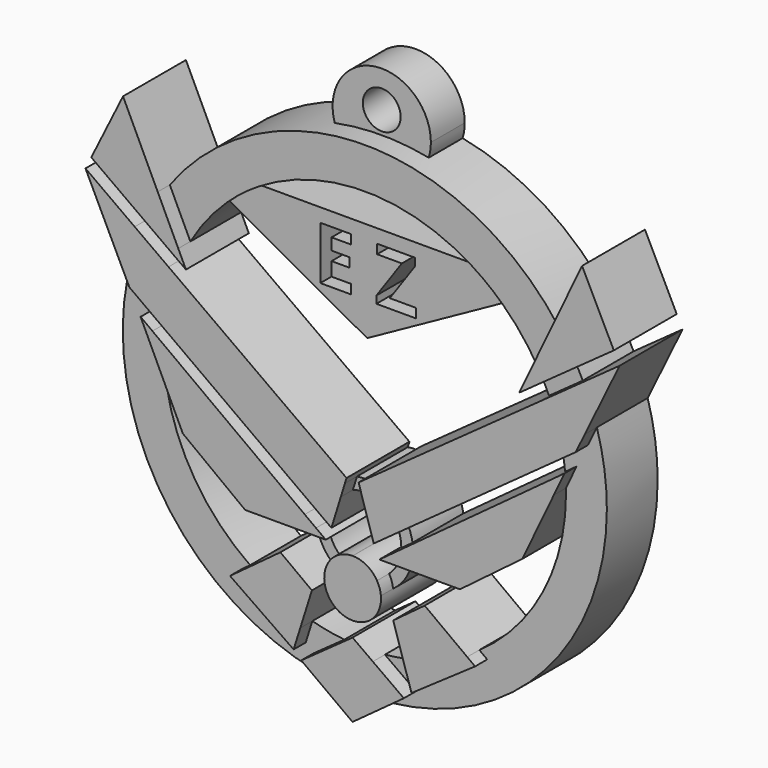
from build123d import *

# Parameters (mm, degrees)
F1_DEPTH = 1.524
F2_DEPTH = 0.254
F3_DEPTH = 5.08
F4_DEPTH = 5.08
F0_R     = 1.5875
F5_DEPTH = 5.08
F6_DEPTH = 1.524


# Not quite as in the source:
# - after a boolean that leaves OpenCascade's solid faulty, fix() repairs it
# - ends of sketch curves that miss each other by under 0.0002 mm in the source are joined
# - a feature names something its author has since deleted; it is built from what else it names


with BuildPart() as f1:
    # F0 (on Front) → F1 (new body)
    with BuildSketch(Plane.XZ):
        with BuildLine():
            Line((-29.3892786764, 17.9176513211), (-25.2442078939, 14.9377645788))
            ThreePointArc((-25.2442078939, 14.9377645788), (-24.5641804468, 16.083185728), (-23.8106040275, 17.1816162074))
            Line((-23.8106040275, 17.1816162074), (-26.7234016986, 23.3000394668))
            Line((-26.7234016986, 23.3000394668), (-29.3892786764, 17.9176513211))
        make_face()
        with BuildLine():
            ThreePointArc((-23.8106040275, 17.1816162074), (-24.5641804468, 16.083185728), (-25.2442078939, 14.9377645788))
            Line((-25.2442078939, 14.9377645788), (-22.4329405216, 12.9167476141))
            ThreePointArc((-22.4329405216, 12.9167476141), (-22.2620008814, 13.2378637775), (-22.084188419, 13.5552258408))
            Line((-22.084188419, 13.5552258408), (-23.8106040275, 17.1816162074))
        make_face()
        with BuildLine():
            ThreePointArc((-22.084188419, 13.5552258408), (-22.2620008814, 13.2378637775), (-22.4329405216, 12.9167476141))
            Line((-22.4329405216, 12.9167476141), (-21.4406050886, 12.2033587829))
            Line((-21.4406050886, 12.2033587829), (-22.084188419, 13.5552258408))
        make_face()
        with BuildLine():
            ThreePointArc((-25.7430354928, 13.9707437059), (-26.401196412, 12.4512059686), (-26.9335086266, 10.8831452437))
            Line((-26.9335086266, 10.8831452437), (-26.1902267417, 9.3535226814))
            Line((-26.1902267417, 9.3535226814), (-24.1110498022, 7.849707391))
            ThreePointArc((-24.1110498022, 7.849707391), (-23.6368154324, 9.9281026338), (-22.9046772821, 11.9302511677))
            Line((-22.9046772821, 11.9302511677), (-25.7430354928, 13.9707437059))
        make_face()
        with BuildLine():
            Line((-29.8784934974, 16.9437198329), (-26.9335086266, 10.8831452437))
            ThreePointArc((-26.9335086266, 10.8831452437), (-26.401196412, 12.4512059686), (-25.7430354928, 13.9707437059))
            Line((-25.7430354928, 13.9707437059), (-29.8784934974, 16.9437198329))
        make_face()
        with BuildLine():
            ThreePointArc((-22.9046772821, 11.9302511677), (-23.6368154324, 9.9281026338), (-24.1110498022, 7.849707391))
            Line((-24.1110498022, 7.849707391), (-11.1208236013, -1.5457896518))
            ThreePointArc((-11.1208236013, -1.5457896518), (-9.886951438, -0.0314606923), (-8.0895618793, 0.7334075888))
            Line((-8.0895618793, 0.7334075888), (-7.9511925062, 1.180207713))
            Line((-7.9511925062, 1.180207713), (-22.9046772821, 11.9302511677))
        make_face()
        with BuildLine():
            ThreePointArc((-8.0895618793, 0.7334075888), (-9.886951438, -0.0314606923), (-11.1208236013, -1.5457896518))
            Line((-11.1208236013, -1.5457896518), (-10.2965646805, -2.1419549635))
            ThreePointArc((-10.2965646805, -2.1419549635), (-9.5580579554, -1.0532702062), (-8.4321576163, -0.3728474624))
            Line((-8.4321576163, -0.3728474624), (-8.0895618793, 0.7334075888))
        make_face()
        with BuildLine():
            ThreePointArc((-8.4321576163, -0.3728474624), (-9.5580579554, -1.0532702062), (-10.2965646805, -2.1419549635))
            Line((-10.2965646805, -2.1419549635), (-9.2209577128, -2.9199138634))
            Line((-9.2209577128, -2.9199138634), (-8.4321576163, -0.3728474624))
        make_face()
        with BuildLine():
            ThreePointArc((-24.2536135862, 6.7439211254), (-24.3005868215, 6.1366695), (-24.3256460235, 5.5281195367))
            Line((-24.3256460235, 5.5281195367), (-21.7045924914, 0))
            Line((-21.7045924914, 0), (-16.4677212918, -3.9508687748))
            Line((-16.4677212918, -3.9508687748), (-11.4556599361, -3.9508687748))
            ThreePointArc((-11.4556599361, -3.9508687748), (-11.5106514951, -3.3027910164), (-11.4616861743, -2.6542301095))
            Line((-11.4616861743, -2.6542301095), (-24.2536135862, 6.7439211254))
        make_face()
        with BuildLine():
            ThreePointArc((-17.0661091722, -8.7456602207), (-14.5563398729, -10.1858082926), (-11.8376665018, -11.1766581835))
            Line((-11.8376665018, -11.1766581835), (-10.8605655167, -8.0768892639))
            Line((-10.8605655167, -8.0768892639), (-13.5054501714, -6.1196745536))
            Line((-13.5054501714, -6.1196745536), (-17.0661091722, -8.7456602207))
        make_face()
        with BuildLine():
            Line((-7.4453192851, -10.4538336357), (-9.147168429, -11.6738428354))
            ThreePointArc((-9.147168429, -11.6738428354), (-7.4437042085, -11.7611295901), (-5.7401185733, -11.676245483))
            Line((-5.7401185733, -11.676245483), (-7.4453192851, -10.4538336357))
        make_face()
        with BuildLine():
            Line((-9.147168429, -11.6738428354), (-11.7522682075, -13.541367761))
            Line((-11.7522682075, -13.541367761), (-9.6607773298, -15.0707744806))
            ThreePointArc((-9.6607773298, -15.0707744806), (-7.4477977116, -15.1933278019), (-5.2346278181, -15.0742600496))
            Line((-5.2346278181, -15.0742600496), (-3.1383703627, -13.541367761))
            Line((-3.1383703627, -13.541367761), (-5.7401185733, -11.676245483))
            ThreePointArc((-5.7401185733, -11.676245483), (-7.4437042085, -11.7611295901), (-9.147168429, -11.6738428354))
        make_face()
        with BuildLine():
            Line((-12.3945986384, -12.9434775331), (-11.8376665018, -11.1766581835))
            ThreePointArc((-11.8376665018, -11.1766581835), (-14.5563398729, -10.1858082926), (-17.0661091722, -8.7456602207))
            Line((-17.0661091722, -8.7456602207), (-17.7372660576, -9.2406383585))
            Line((-17.7372660576, -9.2406383585), (-12.3945986384, -12.9434775331))
        make_face()
        with BuildLine():
            ThreePointArc((2.1885836534, -8.7553310948), (-0.3266501697, -10.194820497), (-3.0508548241, -11.183374959))
            Line((-3.0508548241, -11.183374959), (-2.4960399319, -12.9434775331))
            Line((-2.4960399319, -12.9434775331), (2.8466274874, -9.2406383585))
            Line((2.8466274874, -9.2406383585), (2.1885836534, -8.7553310948))
        make_face()
        with BuildLine():
            Line((-4.0300730536, -8.0768892639), (-3.0508548241, -11.183374959))
            ThreePointArc((-3.0508548241, -11.183374959), (-0.3266501697, -10.194820497), (2.1885836534, -8.7553310948))
            Line((2.1885836534, -8.7553310948), (-1.3851883989, -6.1196745536))
            Line((-1.3851883989, -6.1196745536), (-4.0300730536, -8.0768892639))
        make_face()
        with BuildLine():
            ThreePointArc((-5.2346278181, -15.0742600496), (-7.4477977116, -15.1933278019), (-9.6607773298, -15.0707744806))
            Line((-9.6607773298, -15.0707744806), (-7.4453192851, -16.690832429))
            Line((-7.4453192851, -16.690832429), (-5.2346278181, -15.0742600496))
        make_face()
        with BuildLine():
            Line((6.8139539211, 0), (9.4607287146, 5.5823687939))
            ThreePointArc((9.4607287146, 5.5823687939), (9.4348160904, 6.1730653057), (9.3882543596, 6.7624937054))
            Line((9.3882543596, 6.7624937054), (-3.4220459658, -2.6491559973))
            ThreePointArc((-3.4220459658, -2.6491559973), (-3.3847096309, -2.9655419621), (-3.3722387063, -3.2838791366))
            ThreePointArc((-3.3722387063, -3.2838791366), (-3.3860209225, -3.61850732), (-3.4272742123, -3.9508687748))
            Line((-3.4272742123, -3.9508687748), (1.5770827215, -3.9508687748))
            Line((1.5770827215, -3.9508687748), (6.8139539211, 0))
        make_face()
        with BuildLine():
            ThreePointArc((-3.3722387063, -3.2838791366), (-3.3847096309, -2.9655419621), (-3.4220459658, -2.6491559973))
            Line((-3.4220459658, -2.6491559973), (-4.3670525152, -3.343446559))
            ThreePointArc((-4.3670525152, -3.343446559), (-4.3882256797, -3.6489683665), (-4.4396846069, -3.9508687748))
            Line((-4.4396846069, -3.9508687748), (-3.4272742123, -3.9508687748))
            ThreePointArc((-3.4272742123, -3.9508687748), (-3.3860209225, -3.61850732), (-3.3722387063, -3.2838791366))
        make_face()
        with BuildLine():
            ThreePointArc((-4.4396846069, -3.9508687748), (-4.3882256797, -3.6489683665), (-4.3670525152, -3.343446559))
            Line((-4.3670525152, -3.343446559), (-5.1938215998, -3.9508687748))
            Line((-5.1938215998, -3.9508687748), (-4.4396846069, -3.9508687748))
        make_face()
        with BuildLine():
            Line((-3.7640746818, -1.5416378495), (9.2446181115, 7.8672156054))
            ThreePointArc((9.2446181115, 7.8672156054), (8.7684283615, 9.9443494969), (8.034603349, 11.9450350624))
            Line((8.034603349, 11.9450350624), (-6.9394460641, 1.180207713))
            Line((-6.9394460641, 1.180207713), (-6.8014791203, 0.7347070487))
            ThreePointArc((-6.8014791203, 0.7347070487), (-5.0011023909, -0.027617519), (-3.7640746818, -1.5416378495))
        make_face()
        with BuildLine():
            ThreePointArc((-3.7640746818, -1.5416378495), (-5.0011023909, -0.027617519), (-6.8014791203, 0.7347070487))
            Line((-6.8014791203, 0.7347070487), (-6.4593837101, -0.3699324273))
            ThreePointArc((-6.4593837101, -0.3699324273), (-5.3298655428, -1.0485464698), (-4.5881010795, -2.1376349833))
            Line((-4.5881010795, -2.1376349833), (-3.7640746818, -1.5416378495))
        make_face()
        with BuildLine():
            ThreePointArc((-4.5881010795, -2.1376349833), (-5.3298655428, -1.0485464698), (-6.4593837101, -0.3699324273))
            Line((-6.4593837101, -0.3699324273), (-5.6696808574, -2.9199138634))
            Line((-5.6696808574, -2.9199138634), (-4.5881010795, -2.1376349833))
        make_face()
        with BuildLine():
            Line((11.2995881714, 9.3535226814), (12.0596972292, 10.9177743984))
            ThreePointArc((12.0596972292, 10.9177743984), (11.5282255807, 12.4755284527), (10.8724863967, 13.9851860064))
            Line((10.8724863967, 13.9851860064), (8.034603349, 11.9450350624))
            ThreePointArc((8.034603349, 11.9450350624), (8.7684283615, 9.9443494969), (9.2446181115, 7.8672156054))
            Line((9.2446181115, 7.8672156054), (11.2995881714, 9.3535226814))
        make_face()
        with BuildLine():
            ThreePointArc((10.8724863967, 13.9851860064), (11.5282255807, 12.4755284527), (12.0596972292, 10.9177743984))
            Line((12.0596972292, 10.9177743984), (14.9878549272, 16.9437198329))
            Line((14.9878549272, 16.9437198329), (10.8724863967, 13.9851860064))
        make_face()
        with BuildLine():
            ThreePointArc((8.9305917122, 17.2039369907), (9.6888499732, 16.101563469), (10.3729570975, 14.9517024278))
            Line((10.3729570975, 14.9517024278), (14.4986401061, 17.9176513211))
            Line((14.4986401061, 17.9176513211), (11.8327631283, 23.3000394668))
            Line((11.8327631283, 23.3000394668), (8.9305917122, 17.2039369907))
        make_face()
        with BuildLine():
            Line((7.5620096779, 12.9309154766), (10.3729570975, 14.9517024278))
            ThreePointArc((10.3729570975, 14.9517024278), (9.6888499732, 16.101563469), (8.9305917122, 17.2039369907))
            Line((8.9305917122, 17.2039369907), (7.2058000477, 13.5809577696))
            ThreePointArc((7.2058000477, 13.5809577696), (7.3874695305, 13.2578899867), (7.5620096779, 12.9309154766))
        make_face()
        with BuildLine():
            Line((6.5499665184, 12.2033587829), (7.5620096779, 12.9309154766))
            ThreePointArc((7.5620096779, 12.9309154766), (7.3874695305, 13.2578899867), (7.2058000477, 13.5809577696))
            Line((7.2058000477, 13.5809577696), (6.5499665184, 12.2033587829))
        make_face()
        with BuildLine():
            ThreePointArc((-7.4453190455, -4.409928668), (-8.6202773785, -4.7259875354), (-9.4878146698, -5.5790990992))
            ThreePointArc((-9.4878146698, -5.5790990992), (-7.438916562, -6.3588696494), (-5.3913148142, -5.5757013089))
            ThreePointArc((-5.3913148142, -5.5757013089), (-6.258544157, -4.7250028045), (-7.4317876868, -4.409924563))
            ThreePointArc((-7.4317876868, -4.409924563), (-7.4385532966, -4.4098999663), (-7.4453190455, -4.409928668))
        make_face()
        with BuildLine():
            ThreePointArc((-9.4878146698, -5.5790990992), (-9.707994461, -6.0658997758), (-9.8146467685, -6.5894256344))
            ThreePointArc((-9.8146467685, -6.5894256344), (-7.4380963903, -7.3531061085), (-5.0628144394, -6.5854895244))
            ThreePointArc((-5.0628144394, -6.5854895244), (-5.1703309798, -6.0621390473), (-5.3913148142, -5.5757013089))
            ThreePointArc((-5.3913148142, -5.5757013089), (-7.438916562, -6.3588696494), (-9.4878146698, -5.5790990992))
        make_face()
        with BuildLine():
            ThreePointArc((-5.0628144394, -6.5854895244), (-7.4380963903, -7.3531061085), (-9.8146467685, -6.5894256344))
            ThreePointArc((-9.8146467685, -6.5894256344), (-9.2016251543, -8.4118856878), (-7.4453190919, -9.1945383314))
            ThreePointArc((-7.4453190919, -9.1945383314), (-7.4385533198, -9.1945670332), (-7.4317874936, -9.1945766005))
            ThreePointArc((-7.4317874936, -9.1945766005), (-5.6741540842, -8.410420721), (-5.0628144394, -6.5854895244))
        make_face()
        with BuildLine():
            Line((-25.2487384332, 7.4750332955), (-24.3256460235, 5.5281195367))
            ThreePointArc((-24.3256460235, 5.5281195367), (-24.3005868215, 6.1366695), (-24.2536135862, 6.7439211254))
            Line((-24.2536135862, 6.7439211254), (-25.2487384332, 7.4750332955))
        make_face()
        with BuildLine():
            ThreePointArc((9.3882543596, 6.7624937054), (9.4348160904, 6.1730653057), (9.4607287146, 5.5823687939))
            Line((9.4607287146, 5.5823687939), (10.3580998629, 7.4750332955))
            Line((10.3580998629, 7.4750332955), (9.3882543596, 6.7624937054))
        make_face()
        with BuildLine():
            Line((-10.5157649287, -3.349192693), (-11.4616861743, -2.6542301095))
            ThreePointArc((-11.4616861743, -2.6542301095), (-11.5106514951, -3.3027910164), (-11.4556599361, -3.9508687748))
            Line((-11.4556599361, -3.9508687748), (-10.4432495415, -3.9508687748))
            ThreePointArc((-10.4432495415, -3.9508687748), (-10.4943659501, -3.6518215405), (-10.5157649287, -3.349192693))
        make_face()
        with BuildLine():
            Line((-9.6968169705, -3.9508687748), (-10.5157649287, -3.349192693))
            ThreePointArc((-10.5157649287, -3.349192693), (-10.4943659501, -3.6518215405), (-10.4432495415, -3.9508687748))
            Line((-10.4432495415, -3.9508687748), (-9.6968169705, -3.9508687748))
        make_face()
    extrude(amount=F1_DEPTH)

    # F0 (on Front) → F2 (join)
    with BuildSketch(Plane.XZ):
        with BuildLine():
            ThreePointArc((-11.3830292088, 25.0801688798), (-18.3370431386, 22.2955642053), (-23.8106040275, 17.1816162074))
            Line((-23.8106040275, 17.1816162074), (-22.084188419, 13.5552258408))
            ThreePointArc((-22.084188419, 13.5552258408), (-20.6821639434, 15.6245126242), (-18.9902364597, 17.4643500659))
            ThreePointArc((-18.9902364597, 17.4643500659), (-17.7354816115, 18.5308685342), (-16.3828742663, 19.4701899605))
            ThreePointArc((-16.3828742663, 19.4701899605), (-7.4317874936, 22.0356257085), (1.5192992791, 19.4701899605))
            ThreePointArc((1.5192992791, 19.4701899605), (2.8719066243, 18.5308685342), (4.1266614725, 17.4643500659))
            ThreePointArc((4.1266614725, 17.4643500659), (5.8093705413, 15.6361493332), (7.2058000477, 13.5809577696))
            Line((7.2058000477, 13.5809577696), (8.9305917122, 17.2039369907))
            ThreePointArc((8.9305917122, 17.2039369907), (3.4617682126, 22.3029946988), (-3.4805457784, 25.0801688798))
            ThreePointArc((-3.4805457784, 25.0801688798), (-7.4317874936, 22.1422606566), (-11.3830292088, 25.0801688798))
        make_face()
        with BuildLine():
            Line((8.034603349, 11.9450350624), (10.8724863967, 13.9851860064))
            ThreePointArc((10.8724863967, 13.9851860064), (10.6291881839, 14.4717862965), (10.3729570975, 14.9517024278))
            Line((10.3729570975, 14.9517024278), (7.5620096779, 12.9309154766))
            ThreePointArc((7.5620096779, 12.9309154766), (7.806281725, 12.4417982834), (8.034603349, 11.9450350624))
        make_face()
        with BuildLine():
            Line((7.5620096779, 12.9309154766), (10.3729570975, 14.9517024278))
            ThreePointArc((10.3729570975, 14.9517024278), (9.6888499732, 16.101563469), (8.9305917122, 17.2039369907))
            Line((8.9305917122, 17.2039369907), (7.2058000477, 13.5809577696))
            ThreePointArc((7.2058000477, 13.5809577696), (7.3874695305, 13.2578899867), (7.5620096779, 12.9309154766))
        make_face()
        with BuildLine():
            Line((11.2995881714, 9.3535226814), (12.0596972292, 10.9177743984))
            ThreePointArc((12.0596972292, 10.9177743984), (11.5282255807, 12.4755284527), (10.8724863967, 13.9851860064))
            Line((10.8724863967, 13.9851860064), (8.034603349, 11.9450350624))
            ThreePointArc((8.034603349, 11.9450350624), (8.7684283615, 9.9443494969), (9.2446181115, 7.8672156054))
            Line((9.2446181115, 7.8672156054), (11.2995881714, 9.3535226814))
        make_face()
        with BuildLine():
            ThreePointArc((-3.0508548241, -11.183374959), (-4.3855024026, -11.4842878255), (-5.7401185733, -11.676245483))
            Line((-5.7401185733, -11.676245483), (-3.1383703627, -13.541367761))
            Line((-3.1383703627, -13.541367761), (-5.2346278181, -15.0742600496))
            ThreePointArc((-5.2346278181, -15.0742600496), (7.7009917694, -8.4396269337), (12.8987925706, 5.1372459583))
            ThreePointArc((12.8987925706, 5.1372459583), (12.6879251842, 8.0578019858), (12.0596972292, 10.9177743984))
            Line((12.0596972292, 10.9177743984), (11.2995881714, 9.3535226814))
            Line((11.2995881714, 9.3535226814), (9.2446181115, 7.8672156054))
            ThreePointArc((9.2446181115, 7.8672156054), (9.3255422669, 7.3160386241), (9.3882543596, 6.7624937054))
            Line((9.3882543596, 6.7624937054), (10.3580998629, 7.4750332955))
            Line((10.3580998629, 7.4750332955), (9.4607287146, 5.5823687939))
            ThreePointArc((9.4607287146, 5.5823687939), (9.4651263075, 5.3598266852), (9.4665922566, 5.1372459583))
            ThreePointArc((9.4665922566, 5.1372459583), (7.5369119015, -2.7045189324), (2.1885836534, -8.7553310948))
            Line((2.1885836534, -8.7553310948), (2.8466274874, -9.2406383585))
            Line((2.8466274874, -9.2406383585), (-2.4960399319, -12.9434775331))
            Line((-2.4960399319, -12.9434775331), (-3.0508548241, -11.183374959))
        make_face()
        with BuildLine():
            Line((-9.6607773298, -15.0707744806), (-11.7522682075, -13.541367761))
            Line((-11.7522682075, -13.541367761), (-9.147168429, -11.6738428354))
            ThreePointArc((-9.147168429, -11.6738428354), (-10.5024965272, -11.4797930142), (-11.8376665018, -11.1766581835))
            Line((-11.8376665018, -11.1766581835), (-12.3945986384, -12.9434775331))
            Line((-12.3945986384, -12.9434775331), (-17.7372660576, -9.2406383585))
            Line((-17.7372660576, -9.2406383585), (-17.0661091722, -8.7456602207))
            ThreePointArc((-17.0661091722, -8.7456602207), (-22.4940344519, -2.5232993714), (-24.3256460235, 5.5281195367))
            Line((-24.3256460235, 5.5281195367), (-25.2487384332, 7.4750332955))
            Line((-25.2487384332, 7.4750332955), (-24.2536135862, 6.7439211254))
            ThreePointArc((-24.2536135862, 6.7439211254), (-24.1914540127, 7.2979903555), (-24.1110498022, 7.849707391))
            Line((-24.1110498022, 7.849707391), (-26.1902267417, 9.3535226814))
            Line((-26.1902267417, 9.3535226814), (-26.9335086266, 10.8831452437))
            ThreePointArc((-26.9335086266, 10.8831452437), (-24.3568410259, -6.1266365285), (-9.6607773298, -15.0707744806))
        make_face()
        with BuildLine():
            ThreePointArc((-23.8106040275, 17.1816162074), (-24.5641804468, 16.083185728), (-25.2442078939, 14.9377645788))
            Line((-25.2442078939, 14.9377645788), (-22.4329405216, 12.9167476141))
            ThreePointArc((-22.4329405216, 12.9167476141), (-22.2620008814, 13.2378637775), (-22.084188419, 13.5552258408))
            Line((-22.084188419, 13.5552258408), (-23.8106040275, 17.1816162074))
        make_face()
        with BuildLine():
            ThreePointArc((-25.2442078939, 14.9377645788), (-25.5000922564, 14.4575919146), (-25.7430354928, 13.9707437059))
            Line((-25.7430354928, 13.9707437059), (-22.9046772821, 11.9302511677))
            ThreePointArc((-22.9046772821, 11.9302511677), (-22.6767904521, 12.427316121), (-22.4329405216, 12.9167476141))
            Line((-22.4329405216, 12.9167476141), (-25.2442078939, 14.9377645788))
        make_face()
        with BuildLine():
            ThreePointArc((-25.7430354928, 13.9707437059), (-26.401196412, 12.4512059686), (-26.9335086266, 10.8831452437))
            Line((-26.9335086266, 10.8831452437), (-26.1902267417, 9.3535226814))
            Line((-26.1902267417, 9.3535226814), (-24.1110498022, 7.849707391))
            ThreePointArc((-24.1110498022, 7.849707391), (-23.6368154324, 9.9281026338), (-22.9046772821, 11.9302511677))
            Line((-22.9046772821, 11.9302511677), (-25.7430354928, 13.9707437059))
        make_face()
        with BuildLine():
            Line((-9.147168429, -11.6738428354), (-11.7522682075, -13.541367761))
            Line((-11.7522682075, -13.541367761), (-9.6607773298, -15.0707744806))
            ThreePointArc((-9.6607773298, -15.0707744806), (-7.4477977116, -15.1933278019), (-5.2346278181, -15.0742600496))
            Line((-5.2346278181, -15.0742600496), (-3.1383703627, -13.541367761))
            Line((-3.1383703627, -13.541367761), (-5.7401185733, -11.676245483))
            ThreePointArc((-5.7401185733, -11.676245483), (-7.4437042085, -11.7611295901), (-9.147168429, -11.6738428354))
        make_face()
        with BuildLine():
            ThreePointArc((-6.8014791203, 0.7347070487), (-7.4455722426, 0.7853471606), (-8.0895618793, 0.7334075888))
            Line((-8.0895618793, 0.7334075888), (-8.4321576163, -0.3728474624))
            ThreePointArc((-8.4321576163, -0.3728474624), (-7.4460107771, -0.208890923), (-6.4593837101, -0.3699324273))
            Line((-6.4593837101, -0.3699324273), (-6.8014791203, 0.7347070487))
        make_face()
        with BuildLine():
            Line((-10.2965646805, -2.1419549635), (-11.1208236013, -1.5457896518))
            ThreePointArc((-11.1208236013, -1.5457896518), (-11.3309434235, -2.0878050425), (-11.4616861743, -2.6542301095))
            Line((-11.4616861743, -2.6542301095), (-10.5157649287, -3.349192693))
            ThreePointArc((-10.5157649287, -3.349192693), (-10.4669898995, -2.7345297103), (-10.2965646805, -2.1419549635))
        make_face()
        with BuildLine():
            Line((-10.4432495415, -3.9508687748), (-11.4556599361, -3.9508687748))
            ThreePointArc((-11.4556599361, -3.9508687748), (-10.8969160491, -5.4329468163), (-9.8146467685, -6.5894256344))
            ThreePointArc((-9.8146467685, -6.5894256344), (-9.707994461, -6.0658997758), (-9.4878146698, -5.5790990992))
            ThreePointArc((-9.4878146698, -5.5790990992), (-10.0935771361, -4.8401199208), (-10.4432495415, -3.9508687748))
        make_face()
        with BuildLine():
            ThreePointArc((-5.3913148142, -5.5757013089), (-5.1703309798, -6.0621390473), (-5.0628144394, -6.5854895244))
            ThreePointArc((-5.0628144394, -6.5854895244), (-3.984239137, -5.43008381), (-3.4272742123, -3.9508687748))
            Line((-3.4272742123, -3.9508687748), (-4.4396846069, -3.9508687748))
            ThreePointArc((-4.4396846069, -3.9508687748), (-4.7880671207, -4.8379196269), (-5.3913148142, -5.5757013089))
        make_face()
        with BuildLine():
            ThreePointArc((-3.4220459658, -2.6491559973), (-3.553423398, -2.0831560704), (-3.7640746818, -1.5416378495))
            Line((-3.7640746818, -1.5416378495), (-4.5881010795, -2.1376349833))
            ThreePointArc((-4.5881010795, -2.1376349833), (-4.4223902666, -2.7001425618), (-4.3664755037, -3.2838791366))
            ThreePointArc((-4.3664755037, -3.2838791366), (-4.3666197599, -3.3136642451), (-4.3670525152, -3.343446559))
            Line((-4.3670525152, -3.343446559), (-3.4220459658, -2.6491559973))
        make_face()
        with BuildLine():
            ThreePointArc((-3.4805457784, 25.0801688798), (-7.4317874936, 25.4678260225), (-11.3830292088, 25.0801688798))
            ThreePointArc((-11.3830292088, 25.0801688798), (-7.4317874936, 22.1422606566), (-3.4805457784, 25.0801688798))
        make_face()
    extrude(amount=F2_DEPTH)

    # F0 (on Front) → F3 (join)
    with BuildSketch(Plane.XZ):
        with BuildLine():
            ThreePointArc((-11.3830292088, 25.0801688798), (-18.3370431386, 22.2955642053), (-23.8106040275, 17.1816162074))
            Line((-23.8106040275, 17.1816162074), (-22.084188419, 13.5552258408))
            ThreePointArc((-22.084188419, 13.5552258408), (-20.6821639434, 15.6245126242), (-18.9902364597, 17.4643500659))
            ThreePointArc((-18.9902364597, 17.4643500659), (-17.7354816115, 18.5308685342), (-16.3828742663, 19.4701899605))
            ThreePointArc((-16.3828742663, 19.4701899605), (-7.4317874936, 22.0356257085), (1.5192992791, 19.4701899605))
            ThreePointArc((1.5192992791, 19.4701899605), (2.8719066243, 18.5308685342), (4.1266614725, 17.4643500659))
            ThreePointArc((4.1266614725, 17.4643500659), (5.8093705413, 15.6361493332), (7.2058000477, 13.5809577696))
            Line((7.2058000477, 13.5809577696), (8.9305917122, 17.2039369907))
            ThreePointArc((8.9305917122, 17.2039369907), (3.4617682126, 22.3029946988), (-3.4805457784, 25.0801688798))
            ThreePointArc((-3.4805457784, 25.0801688798), (-7.4317874936, 22.1422606566), (-11.3830292088, 25.0801688798))
        make_face()
        with BuildLine():
            Line((7.5620096779, 12.9309154766), (10.3729570975, 14.9517024278))
            ThreePointArc((10.3729570975, 14.9517024278), (9.6888499732, 16.101563469), (8.9305917122, 17.2039369907))
            Line((8.9305917122, 17.2039369907), (7.2058000477, 13.5809577696))
            ThreePointArc((7.2058000477, 13.5809577696), (7.3874695305, 13.2578899867), (7.5620096779, 12.9309154766))
        make_face()
        with BuildLine():
            Line((8.034603349, 11.9450350624), (10.8724863967, 13.9851860064))
            ThreePointArc((10.8724863967, 13.9851860064), (10.6291881839, 14.4717862965), (10.3729570975, 14.9517024278))
            Line((10.3729570975, 14.9517024278), (7.5620096779, 12.9309154766))
            ThreePointArc((7.5620096779, 12.9309154766), (7.806281725, 12.4417982834), (8.034603349, 11.9450350624))
        make_face()
        with BuildLine():
            Line((11.2995881714, 9.3535226814), (12.0596972292, 10.9177743984))
            ThreePointArc((12.0596972292, 10.9177743984), (11.5282255807, 12.4755284527), (10.8724863967, 13.9851860064))
            Line((10.8724863967, 13.9851860064), (8.034603349, 11.9450350624))
            ThreePointArc((8.034603349, 11.9450350624), (8.7684283615, 9.9443494969), (9.2446181115, 7.8672156054))
            Line((9.2446181115, 7.8672156054), (11.2995881714, 9.3535226814))
        make_face()
        with BuildLine():
            ThreePointArc((-3.0508548241, -11.183374959), (-4.3855024026, -11.4842878255), (-5.7401185733, -11.676245483))
            Line((-5.7401185733, -11.676245483), (-3.1383703627, -13.541367761))
            Line((-3.1383703627, -13.541367761), (-5.2346278181, -15.0742600496))
            ThreePointArc((-5.2346278181, -15.0742600496), (7.7009917694, -8.4396269337), (12.8987925706, 5.1372459583))
            ThreePointArc((12.8987925706, 5.1372459583), (12.6879251842, 8.0578019858), (12.0596972292, 10.9177743984))
            Line((12.0596972292, 10.9177743984), (11.2995881714, 9.3535226814))
            Line((11.2995881714, 9.3535226814), (9.2446181115, 7.8672156054))
            ThreePointArc((9.2446181115, 7.8672156054), (9.3255422669, 7.3160386241), (9.3882543596, 6.7624937054))
            Line((9.3882543596, 6.7624937054), (10.3580998629, 7.4750332955))
            Line((10.3580998629, 7.4750332955), (9.4607287146, 5.5823687939))
            ThreePointArc((9.4607287146, 5.5823687939), (9.4651263075, 5.3598266852), (9.4665922566, 5.1372459583))
            ThreePointArc((9.4665922566, 5.1372459583), (7.5369119015, -2.7045189324), (2.1885836534, -8.7553310948))
            Line((2.1885836534, -8.7553310948), (2.8466274874, -9.2406383585))
            Line((2.8466274874, -9.2406383585), (-2.4960399319, -12.9434775331))
            Line((-2.4960399319, -12.9434775331), (-3.0508548241, -11.183374959))
        make_face()
        with BuildLine():
            Line((-9.147168429, -11.6738428354), (-11.7522682075, -13.541367761))
            Line((-11.7522682075, -13.541367761), (-9.6607773298, -15.0707744806))
            ThreePointArc((-9.6607773298, -15.0707744806), (-7.4477977116, -15.1933278019), (-5.2346278181, -15.0742600496))
            Line((-5.2346278181, -15.0742600496), (-3.1383703627, -13.541367761))
            Line((-3.1383703627, -13.541367761), (-5.7401185733, -11.676245483))
            ThreePointArc((-5.7401185733, -11.676245483), (-7.4437042085, -11.7611295901), (-9.147168429, -11.6738428354))
        make_face()
        with BuildLine():
            Line((-9.6607773298, -15.0707744806), (-11.7522682075, -13.541367761))
            Line((-11.7522682075, -13.541367761), (-9.147168429, -11.6738428354))
            ThreePointArc((-9.147168429, -11.6738428354), (-10.5024965272, -11.4797930142), (-11.8376665018, -11.1766581835))
            Line((-11.8376665018, -11.1766581835), (-12.3945986384, -12.9434775331))
            Line((-12.3945986384, -12.9434775331), (-17.7372660576, -9.2406383585))
            Line((-17.7372660576, -9.2406383585), (-17.0661091722, -8.7456602207))
            ThreePointArc((-17.0661091722, -8.7456602207), (-22.4940344519, -2.5232993714), (-24.3256460235, 5.5281195367))
            Line((-24.3256460235, 5.5281195367), (-25.2487384332, 7.4750332955))
            Line((-25.2487384332, 7.4750332955), (-24.2536135862, 6.7439211254))
            ThreePointArc((-24.2536135862, 6.7439211254), (-24.1914540127, 7.2979903555), (-24.1110498022, 7.849707391))
            Line((-24.1110498022, 7.849707391), (-26.1902267417, 9.3535226814))
            Line((-26.1902267417, 9.3535226814), (-26.9335086266, 10.8831452437))
            ThreePointArc((-26.9335086266, 10.8831452437), (-24.3568410259, -6.1266365285), (-9.6607773298, -15.0707744806))
        make_face()
        with BuildLine():
            ThreePointArc((-25.7430354928, 13.9707437059), (-26.401196412, 12.4512059686), (-26.9335086266, 10.8831452437))
            Line((-26.9335086266, 10.8831452437), (-26.1902267417, 9.3535226814))
            Line((-26.1902267417, 9.3535226814), (-24.1110498022, 7.849707391))
            ThreePointArc((-24.1110498022, 7.849707391), (-23.6368154324, 9.9281026338), (-22.9046772821, 11.9302511677))
            Line((-22.9046772821, 11.9302511677), (-25.7430354928, 13.9707437059))
        make_face()
        with BuildLine():
            ThreePointArc((-25.2442078939, 14.9377645788), (-25.5000922564, 14.4575919146), (-25.7430354928, 13.9707437059))
            Line((-25.7430354928, 13.9707437059), (-22.9046772821, 11.9302511677))
            ThreePointArc((-22.9046772821, 11.9302511677), (-22.6767904521, 12.427316121), (-22.4329405216, 12.9167476141))
            Line((-22.4329405216, 12.9167476141), (-25.2442078939, 14.9377645788))
        make_face()
        with BuildLine():
            ThreePointArc((-23.8106040275, 17.1816162074), (-24.5641804468, 16.083185728), (-25.2442078939, 14.9377645788))
            Line((-25.2442078939, 14.9377645788), (-22.4329405216, 12.9167476141))
            ThreePointArc((-22.4329405216, 12.9167476141), (-22.2620008814, 13.2378637775), (-22.084188419, 13.5552258408))
            Line((-22.084188419, 13.5552258408), (-23.8106040275, 17.1816162074))
        make_face()
        with BuildLine():
            ThreePointArc((-6.8014791203, 0.7347070487), (-7.4455722426, 0.7853471606), (-8.0895618793, 0.7334075888))
            Line((-8.0895618793, 0.7334075888), (-8.4321576163, -0.3728474624))
            ThreePointArc((-8.4321576163, -0.3728474624), (-7.4460107771, -0.208890923), (-6.4593837101, -0.3699324273))
            Line((-6.4593837101, -0.3699324273), (-6.8014791203, 0.7347070487))
        make_face()
        with BuildLine():
            ThreePointArc((-3.7640746818, -1.5416378495), (-5.0011023909, -0.027617519), (-6.8014791203, 0.7347070487))
            Line((-6.8014791203, 0.7347070487), (-6.4593837101, -0.3699324273))
            ThreePointArc((-6.4593837101, -0.3699324273), (-5.3298655428, -1.0485464698), (-4.5881010795, -2.1376349833))
            Line((-4.5881010795, -2.1376349833), (-3.7640746818, -1.5416378495))
        make_face()
        with BuildLine():
            ThreePointArc((-3.4220459658, -2.6491559973), (-3.553423398, -2.0831560704), (-3.7640746818, -1.5416378495))
            Line((-3.7640746818, -1.5416378495), (-4.5881010795, -2.1376349833))
            ThreePointArc((-4.5881010795, -2.1376349833), (-4.4223902666, -2.7001425618), (-4.3664755037, -3.2838791366))
            ThreePointArc((-4.3664755037, -3.2838791366), (-4.3666197599, -3.3136642451), (-4.3670525152, -3.343446559))
            Line((-4.3670525152, -3.343446559), (-3.4220459658, -2.6491559973))
        make_face()
        with BuildLine():
            ThreePointArc((-5.3913148142, -5.5757013089), (-5.1703309798, -6.0621390473), (-5.0628144394, -6.5854895244))
            ThreePointArc((-5.0628144394, -6.5854895244), (-3.984239137, -5.43008381), (-3.4272742123, -3.9508687748))
            Line((-3.4272742123, -3.9508687748), (-4.4396846069, -3.9508687748))
            ThreePointArc((-4.4396846069, -3.9508687748), (-4.7880671207, -4.8379196269), (-5.3913148142, -5.5757013089))
        make_face()
        with BuildLine():
            ThreePointArc((-9.4878146698, -5.5790990992), (-9.707994461, -6.0658997758), (-9.8146467685, -6.5894256344))
            ThreePointArc((-9.8146467685, -6.5894256344), (-7.4380963903, -7.3531061085), (-5.0628144394, -6.5854895244))
            ThreePointArc((-5.0628144394, -6.5854895244), (-5.1703309798, -6.0621390473), (-5.3913148142, -5.5757013089))
            ThreePointArc((-5.3913148142, -5.5757013089), (-7.438916562, -6.3588696494), (-9.4878146698, -5.5790990992))
        make_face()
        with BuildLine():
            Line((-10.4432495415, -3.9508687748), (-11.4556599361, -3.9508687748))
            ThreePointArc((-11.4556599361, -3.9508687748), (-10.8969160491, -5.4329468163), (-9.8146467685, -6.5894256344))
            ThreePointArc((-9.8146467685, -6.5894256344), (-9.707994461, -6.0658997758), (-9.4878146698, -5.5790990992))
            ThreePointArc((-9.4878146698, -5.5790990992), (-10.0935771361, -4.8401199208), (-10.4432495415, -3.9508687748))
        make_face()
        with BuildLine():
            Line((-10.2965646805, -2.1419549635), (-11.1208236013, -1.5457896518))
            ThreePointArc((-11.1208236013, -1.5457896518), (-11.3309434235, -2.0878050425), (-11.4616861743, -2.6542301095))
            Line((-11.4616861743, -2.6542301095), (-10.5157649287, -3.349192693))
            ThreePointArc((-10.5157649287, -3.349192693), (-10.4669898995, -2.7345297103), (-10.2965646805, -2.1419549635))
        make_face()
        with BuildLine():
            ThreePointArc((-3.3722387063, -3.2838791366), (-3.3847096309, -2.9655419621), (-3.4220459658, -2.6491559973))
            Line((-3.4220459658, -2.6491559973), (-4.3670525152, -3.343446559))
            ThreePointArc((-4.3670525152, -3.343446559), (-4.3882256797, -3.6489683665), (-4.4396846069, -3.9508687748))
            Line((-4.4396846069, -3.9508687748), (-3.4272742123, -3.9508687748))
            ThreePointArc((-3.4272742123, -3.9508687748), (-3.3860209225, -3.61850732), (-3.3722387063, -3.2838791366))
        make_face()
        with BuildLine():
            Line((-10.5157649287, -3.349192693), (-11.4616861743, -2.6542301095))
            ThreePointArc((-11.4616861743, -2.6542301095), (-11.5106514951, -3.3027910164), (-11.4556599361, -3.9508687748))
            Line((-11.4556599361, -3.9508687748), (-10.4432495415, -3.9508687748))
            ThreePointArc((-10.4432495415, -3.9508687748), (-10.4943659501, -3.6518215405), (-10.5157649287, -3.349192693))
        make_face()
        with BuildLine():
            ThreePointArc((-8.0895618793, 0.7334075888), (-9.886951438, -0.0314606923), (-11.1208236013, -1.5457896518))
            Line((-11.1208236013, -1.5457896518), (-10.2965646805, -2.1419549635))
            ThreePointArc((-10.2965646805, -2.1419549635), (-9.5580579554, -1.0532702062), (-8.4321576163, -0.3728474624))
            Line((-8.4321576163, -0.3728474624), (-8.0895618793, 0.7334075888))
        make_face()
        with BuildLine():
            ThreePointArc((-3.4805457784, 25.0801688798), (-7.4317874936, 25.4678260225), (-11.3830292088, 25.0801688798))
            ThreePointArc((-11.3830292088, 25.0801688798), (-7.4317874936, 22.1422606566), (-3.4805457784, 25.0801688798))
        make_face()
    extrude(amount=-F3_DEPTH)

    # F0 (on Front) → F4 (join)
    with BuildSketch(Plane.XZ):
        with BuildLine():
            ThreePointArc((8.9305917122, 17.2039369907), (9.6888499732, 16.101563469), (10.3729570975, 14.9517024278))
            Line((10.3729570975, 14.9517024278), (14.4986401061, 17.9176513211))
            Line((14.4986401061, 17.9176513211), (11.8327631283, 23.3000394668))
            Line((11.8327631283, 23.3000394668), (8.9305917122, 17.2039369907))
        make_face()
        with BuildLine():
            Line((6.5499665184, 12.2033587829), (7.5620096779, 12.9309154766))
            ThreePointArc((7.5620096779, 12.9309154766), (7.3874695305, 13.2578899867), (7.2058000477, 13.5809577696))
            Line((7.2058000477, 13.5809577696), (6.5499665184, 12.2033587829))
        make_face()
        with BuildLine():
            ThreePointArc((10.8724863967, 13.9851860064), (11.5282255807, 12.4755284527), (12.0596972292, 10.9177743984))
            Line((12.0596972292, 10.9177743984), (14.9878549272, 16.9437198329))
            Line((14.9878549272, 16.9437198329), (10.8724863967, 13.9851860064))
        make_face()
        with BuildLine():
            Line((-3.7640746818, -1.5416378495), (9.2446181115, 7.8672156054))
            ThreePointArc((9.2446181115, 7.8672156054), (8.7684283615, 9.9443494969), (8.034603349, 11.9450350624))
            Line((8.034603349, 11.9450350624), (-6.9394460641, 1.180207713))
            Line((-6.9394460641, 1.180207713), (-6.8014791203, 0.7347070487))
            ThreePointArc((-6.8014791203, 0.7347070487), (-5.0011023909, -0.027617519), (-3.7640746818, -1.5416378495))
        make_face()
        with BuildLine():
            ThreePointArc((-3.7640746818, -1.5416378495), (-5.0011023909, -0.027617519), (-6.8014791203, 0.7347070487))
            Line((-6.8014791203, 0.7347070487), (-6.4593837101, -0.3699324273))
            ThreePointArc((-6.4593837101, -0.3699324273), (-5.3298655428, -1.0485464698), (-4.5881010795, -2.1376349833))
            Line((-4.5881010795, -2.1376349833), (-3.7640746818, -1.5416378495))
        make_face()
        with BuildLine():
            ThreePointArc((-4.5881010795, -2.1376349833), (-5.3298655428, -1.0485464698), (-6.4593837101, -0.3699324273))
            Line((-6.4593837101, -0.3699324273), (-5.6696808574, -2.9199138634))
            Line((-5.6696808574, -2.9199138634), (-4.5881010795, -2.1376349833))
        make_face()
        with BuildLine():
            Line((6.8139539211, 0), (9.4607287146, 5.5823687939))
            ThreePointArc((9.4607287146, 5.5823687939), (9.4348160904, 6.1730653057), (9.3882543596, 6.7624937054))
            Line((9.3882543596, 6.7624937054), (-3.4220459658, -2.6491559973))
            ThreePointArc((-3.4220459658, -2.6491559973), (-3.3847096309, -2.9655419621), (-3.3722387063, -3.2838791366))
            ThreePointArc((-3.3722387063, -3.2838791366), (-3.3860209225, -3.61850732), (-3.4272742123, -3.9508687748))
            Line((-3.4272742123, -3.9508687748), (1.5770827215, -3.9508687748))
            Line((1.5770827215, -3.9508687748), (6.8139539211, 0))
        make_face()
        with BuildLine():
            ThreePointArc((-3.3722387063, -3.2838791366), (-3.3847096309, -2.9655419621), (-3.4220459658, -2.6491559973))
            Line((-3.4220459658, -2.6491559973), (-4.3670525152, -3.343446559))
            ThreePointArc((-4.3670525152, -3.343446559), (-4.3882256797, -3.6489683665), (-4.4396846069, -3.9508687748))
            Line((-4.4396846069, -3.9508687748), (-3.4272742123, -3.9508687748))
            ThreePointArc((-3.4272742123, -3.9508687748), (-3.3860209225, -3.61850732), (-3.3722387063, -3.2838791366))
        make_face()
        with BuildLine():
            ThreePointArc((-4.4396846069, -3.9508687748), (-4.3882256797, -3.6489683665), (-4.3670525152, -3.343446559))
            Line((-4.3670525152, -3.343446559), (-5.1938215998, -3.9508687748))
            Line((-5.1938215998, -3.9508687748), (-4.4396846069, -3.9508687748))
        make_face()
        with BuildLine():
            ThreePointArc((-22.9046772821, 11.9302511677), (-23.6368154324, 9.9281026338), (-24.1110498022, 7.849707391))
            Line((-24.1110498022, 7.849707391), (-11.1208236013, -1.5457896518))
            ThreePointArc((-11.1208236013, -1.5457896518), (-9.886951438, -0.0314606923), (-8.0895618793, 0.7334075888))
            Line((-8.0895618793, 0.7334075888), (-7.9511925062, 1.180207713))
            Line((-7.9511925062, 1.180207713), (-22.9046772821, 11.9302511677))
        make_face()
        with BuildLine():
            ThreePointArc((-8.0895618793, 0.7334075888), (-9.886951438, -0.0314606923), (-11.1208236013, -1.5457896518))
            Line((-11.1208236013, -1.5457896518), (-10.2965646805, -2.1419549635))
            ThreePointArc((-10.2965646805, -2.1419549635), (-9.5580579554, -1.0532702062), (-8.4321576163, -0.3728474624))
            Line((-8.4321576163, -0.3728474624), (-8.0895618793, 0.7334075888))
        make_face()
        with BuildLine():
            ThreePointArc((-8.4321576163, -0.3728474624), (-9.5580579554, -1.0532702062), (-10.2965646805, -2.1419549635))
            Line((-10.2965646805, -2.1419549635), (-9.2209577128, -2.9199138634))
            Line((-9.2209577128, -2.9199138634), (-8.4321576163, -0.3728474624))
        make_face()
        with BuildLine():
            ThreePointArc((-24.2536135862, 6.7439211254), (-24.3005868215, 6.1366695), (-24.3256460235, 5.5281195367))
            Line((-24.3256460235, 5.5281195367), (-21.7045924914, 0))
            Line((-21.7045924914, 0), (-16.4677212918, -3.9508687748))
            Line((-16.4677212918, -3.9508687748), (-11.4556599361, -3.9508687748))
            ThreePointArc((-11.4556599361, -3.9508687748), (-11.5106514951, -3.3027910164), (-11.4616861743, -2.6542301095))
            Line((-11.4616861743, -2.6542301095), (-24.2536135862, 6.7439211254))
        make_face()
        with BuildLine():
            ThreePointArc((-17.0661091722, -8.7456602207), (-14.5563398729, -10.1858082926), (-11.8376665018, -11.1766581835))
            Line((-11.8376665018, -11.1766581835), (-10.8605655167, -8.0768892639))
            Line((-10.8605655167, -8.0768892639), (-13.5054501714, -6.1196745536))
            Line((-13.5054501714, -6.1196745536), (-17.0661091722, -8.7456602207))
        make_face()
        with BuildLine():
            Line((-4.0300730536, -8.0768892639), (-3.0508548241, -11.183374959))
            ThreePointArc((-3.0508548241, -11.183374959), (-0.3266501697, -10.194820497), (2.1885836534, -8.7553310948))
            Line((2.1885836534, -8.7553310948), (-1.3851883989, -6.1196745536))
            Line((-1.3851883989, -6.1196745536), (-4.0300730536, -8.0768892639))
        make_face()
        with BuildLine():
            ThreePointArc((-7.4453190455, -4.409928668), (-8.6202773785, -4.7259875354), (-9.4878146698, -5.5790990992))
            ThreePointArc((-9.4878146698, -5.5790990992), (-7.438916562, -6.3588696494), (-5.3913148142, -5.5757013089))
            ThreePointArc((-5.3913148142, -5.5757013089), (-6.258544157, -4.7250028045), (-7.4317876868, -4.409924563))
            ThreePointArc((-7.4317876868, -4.409924563), (-7.4385532966, -4.4098999663), (-7.4453190455, -4.409928668))
        make_face()
        with BuildLine():
            ThreePointArc((-9.4878146698, -5.5790990992), (-9.707994461, -6.0658997758), (-9.8146467685, -6.5894256344))
            ThreePointArc((-9.8146467685, -6.5894256344), (-7.4380963903, -7.3531061085), (-5.0628144394, -6.5854895244))
            ThreePointArc((-5.0628144394, -6.5854895244), (-5.1703309798, -6.0621390473), (-5.3913148142, -5.5757013089))
            ThreePointArc((-5.3913148142, -5.5757013089), (-7.438916562, -6.3588696494), (-9.4878146698, -5.5790990992))
        make_face()
        with BuildLine():
            ThreePointArc((-5.0628144394, -6.5854895244), (-7.4380963903, -7.3531061085), (-9.8146467685, -6.5894256344))
            ThreePointArc((-9.8146467685, -6.5894256344), (-9.2016251543, -8.4118856878), (-7.4453190919, -9.1945383314))
            ThreePointArc((-7.4453190919, -9.1945383314), (-7.4385533198, -9.1945670332), (-7.4317874936, -9.1945766005))
            ThreePointArc((-7.4317874936, -9.1945766005), (-5.6741540842, -8.410420721), (-5.0628144394, -6.5854895244))
        make_face()
        with BuildLine():
            Line((-7.4453192851, -10.4538336357), (-9.147168429, -11.6738428354))
            ThreePointArc((-9.147168429, -11.6738428354), (-7.4437042085, -11.7611295901), (-5.7401185733, -11.676245483))
            Line((-5.7401185733, -11.676245483), (-7.4453192851, -10.4538336357))
        make_face()
        with BuildLine():
            ThreePointArc((-5.2346278181, -15.0742600496), (-7.4477977116, -15.1933278019), (-9.6607773298, -15.0707744806))
            Line((-9.6607773298, -15.0707744806), (-7.4453192851, -16.690832429))
            Line((-7.4453192851, -16.690832429), (-5.2346278181, -15.0742600496))
        make_face()
        with BuildLine():
            ThreePointArc((2.1885836534, -8.7553310948), (-0.3266501697, -10.194820497), (-3.0508548241, -11.183374959))
            Line((-3.0508548241, -11.183374959), (-2.4960399319, -12.9434775331))
            Line((-2.4960399319, -12.9434775331), (2.8466274874, -9.2406383585))
            Line((2.8466274874, -9.2406383585), (2.1885836534, -8.7553310948))
        make_face()
        with BuildLine():
            Line((-12.3945986384, -12.9434775331), (-11.8376665018, -11.1766581835))
            ThreePointArc((-11.8376665018, -11.1766581835), (-14.5563398729, -10.1858082926), (-17.0661091722, -8.7456602207))
            Line((-17.0661091722, -8.7456602207), (-17.7372660576, -9.2406383585))
            Line((-17.7372660576, -9.2406383585), (-12.3945986384, -12.9434775331))
        make_face()
        with BuildLine():
            Line((-29.8784934974, 16.9437198329), (-26.9335086266, 10.8831452437))
            ThreePointArc((-26.9335086266, 10.8831452437), (-26.401196412, 12.4512059686), (-25.7430354928, 13.9707437059))
            Line((-25.7430354928, 13.9707437059), (-29.8784934974, 16.9437198329))
        make_face()
        with BuildLine():
            Line((-29.3892786764, 17.9176513211), (-25.2442078939, 14.9377645788))
            ThreePointArc((-25.2442078939, 14.9377645788), (-24.5641804468, 16.083185728), (-23.8106040275, 17.1816162074))
            Line((-23.8106040275, 17.1816162074), (-26.7234016986, 23.3000394668))
            Line((-26.7234016986, 23.3000394668), (-29.3892786764, 17.9176513211))
        make_face()
        with BuildLine():
            Line((7.5620096779, 12.9309154766), (10.3729570975, 14.9517024278))
            ThreePointArc((10.3729570975, 14.9517024278), (9.6888499732, 16.101563469), (8.9305917122, 17.2039369907))
            Line((8.9305917122, 17.2039369907), (7.2058000477, 13.5809577696))
            ThreePointArc((7.2058000477, 13.5809577696), (7.3874695305, 13.2578899867), (7.5620096779, 12.9309154766))
        make_face()
        with BuildLine():
            Line((11.2995881714, 9.3535226814), (12.0596972292, 10.9177743984))
            ThreePointArc((12.0596972292, 10.9177743984), (11.5282255807, 12.4755284527), (10.8724863967, 13.9851860064))
            Line((10.8724863967, 13.9851860064), (8.034603349, 11.9450350624))
            ThreePointArc((8.034603349, 11.9450350624), (8.7684283615, 9.9443494969), (9.2446181115, 7.8672156054))
            Line((9.2446181115, 7.8672156054), (11.2995881714, 9.3535226814))
        make_face()
        with BuildLine():
            ThreePointArc((9.3882543596, 6.7624937054), (9.4348160904, 6.1730653057), (9.4607287146, 5.5823687939))
            Line((9.4607287146, 5.5823687939), (10.3580998629, 7.4750332955))
            Line((10.3580998629, 7.4750332955), (9.3882543596, 6.7624937054))
        make_face()
        with BuildLine():
            Line((-25.2487384332, 7.4750332955), (-24.3256460235, 5.5281195367))
            ThreePointArc((-24.3256460235, 5.5281195367), (-24.3005868215, 6.1366695), (-24.2536135862, 6.7439211254))
            Line((-24.2536135862, 6.7439211254), (-25.2487384332, 7.4750332955))
        make_face()
        with BuildLine():
            ThreePointArc((-23.8106040275, 17.1816162074), (-24.5641804468, 16.083185728), (-25.2442078939, 14.9377645788))
            Line((-25.2442078939, 14.9377645788), (-22.4329405216, 12.9167476141))
            ThreePointArc((-22.4329405216, 12.9167476141), (-22.2620008814, 13.2378637775), (-22.084188419, 13.5552258408))
            Line((-22.084188419, 13.5552258408), (-23.8106040275, 17.1816162074))
        make_face()
        with BuildLine():
            ThreePointArc((-22.084188419, 13.5552258408), (-22.2620008814, 13.2378637775), (-22.4329405216, 12.9167476141))
            Line((-22.4329405216, 12.9167476141), (-21.4406050886, 12.2033587829))
            Line((-21.4406050886, 12.2033587829), (-22.084188419, 13.5552258408))
        make_face()
        with BuildLine():
            ThreePointArc((-25.7430354928, 13.9707437059), (-26.401196412, 12.4512059686), (-26.9335086266, 10.8831452437))
            Line((-26.9335086266, 10.8831452437), (-26.1902267417, 9.3535226814))
            Line((-26.1902267417, 9.3535226814), (-24.1110498022, 7.849707391))
            ThreePointArc((-24.1110498022, 7.849707391), (-23.6368154324, 9.9281026338), (-22.9046772821, 11.9302511677))
            Line((-22.9046772821, 11.9302511677), (-25.7430354928, 13.9707437059))
        make_face()
        with BuildLine():
            Line((-9.147168429, -11.6738428354), (-11.7522682075, -13.541367761))
            Line((-11.7522682075, -13.541367761), (-9.6607773298, -15.0707744806))
            ThreePointArc((-9.6607773298, -15.0707744806), (-7.4477977116, -15.1933278019), (-5.2346278181, -15.0742600496))
            Line((-5.2346278181, -15.0742600496), (-3.1383703627, -13.541367761))
            Line((-3.1383703627, -13.541367761), (-5.7401185733, -11.676245483))
            ThreePointArc((-5.7401185733, -11.676245483), (-7.4437042085, -11.7611295901), (-9.147168429, -11.6738428354))
        make_face()
        with BuildLine():
            Line((-10.5157649287, -3.349192693), (-11.4616861743, -2.6542301095))
            ThreePointArc((-11.4616861743, -2.6542301095), (-11.5106514951, -3.3027910164), (-11.4556599361, -3.9508687748))
            Line((-11.4556599361, -3.9508687748), (-10.4432495415, -3.9508687748))
            ThreePointArc((-10.4432495415, -3.9508687748), (-10.4943659501, -3.6518215405), (-10.5157649287, -3.349192693))
        make_face()
        with BuildLine():
            Line((-9.6968169705, -3.9508687748), (-10.5157649287, -3.349192693))
            ThreePointArc((-10.5157649287, -3.349192693), (-10.4943659501, -3.6518215405), (-10.4432495415, -3.9508687748))
            Line((-10.4432495415, -3.9508687748), (-9.6968169705, -3.9508687748))
        make_face()
        with BuildLine():
            ThreePointArc((-16.3828742663, 19.4701899605), (-17.7354816115, 18.5308685342), (-18.9902364597, 17.4643500659))
            Line((-18.9902364597, 17.4643500659), (-7.4360714177, 11.0693256116))
            Line((-7.4360714177, 11.0693256116), (4.1266614725, 17.4643500659))
            ThreePointArc((4.1266614725, 17.4643500659), (2.8719066243, 18.5308685342), (1.5192992791, 19.4701899605))
            Line((1.5192992791, 19.4701899605), (-16.3828742663, 19.4701899605))
        make_face()
        Polygon((-8.8048722859, 14.6434810449), (-8.8048722859, 13.8621462646), (-11.3744870444, 13.8621462646), (-11.3744870444, 18.3245445283), (-8.8048722859, 18.3245445283), (-8.8048722859, 17.5490697589), (-10.4280952918, 17.5490697589), (-10.4280952918, 16.5694712782), (-8.9171891605, 16.5694712782), (-8.9171891605, 15.7939965088), (-10.4280952918, 15.7939965088), (-10.4280952918, 14.6434810449), align=None, mode=Mode.SUBTRACT)
        Polygon((-3.341388835, 14.6434810449), (-3.341388835, 13.8621462646), (-6.662061651, 13.8621462646), (-6.662061651, 14.4754940671), (-4.5221810216, 17.5432097481), (-6.6034615425, 17.5432097481), (-6.6034615425, 18.3245445283), (-3.399012275, 18.3245445283), (-3.399012275, 17.7141267313), (-5.535962899, 14.6434810449), align=None, mode=Mode.SUBTRACT)
    extrude(amount=-F4_DEPTH)

    # F0 (on Front) → F5 (join)
    with BuildSketch(Plane.XZ):
        with BuildLine():
            ThreePointArc((-3.3057879766, 26.2682601736), (-8.0322250864, 30.3503364481), (-11.3830292088, 25.0801688798))
            ThreePointArc((-11.3830292088, 25.0801688798), (-7.4317874936, 25.4678260225), (-3.4805457784, 25.0801688798))
            ThreePointArc((-3.4805457784, 25.0801688798), (-3.349711219, 25.6678225807), (-3.3057879766, 26.2682601736))
        make_face()
        with Locations((-7.4317874936, 27.3330934272)):
            Circle(F0_R, mode=Mode.SUBTRACT)
    extrude(amount=-F5_DEPTH)

    add(f1.part.fix(), mode=Mode.REPLACE)

    # F6 (cut): a face of the model
    f6_faces = [f1.faces().sort_by_distance(p)[0] for p in [
        (-7.4317874936, 0, 30.2961092707),
    ]]
    extrude(f6_faces, amount=-F6_DEPTH, mode=Mode.SUBTRACT)


solid = f1.part
